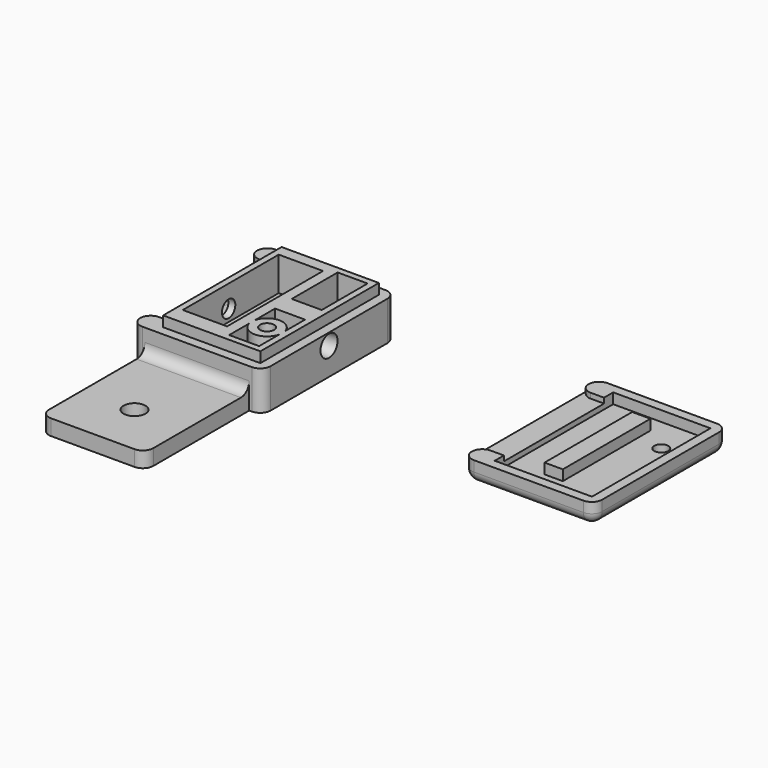
from build123d import *

# Parameters (mm, degrees)
F0_W      = 2
F0_H      = 24
F0_W_2    = 20
F0_H_2    = 25
F1_DEPTH  = 3
F2_W      = 8.5
F2_H      = 26
F2_R      = 1.35
F2_W_2    = 5.75
F2_H_2    = 4
F3_DEPTH  = 4.5
F2_R_2    = 2.1
F4_DEPTH  = 25
F5_W      = 18.65
F5_H      = 28.4
F5_R      = 1.35
F5_W_2    = 8.5
F5_H_2    = 26
F5_W_3    = 5.75
F5_H_3    = 11
F6_DEPTH  = 2
F8_R      = 1.1
F7_R      = 1.1
F9_DEPTH  = 11
F9_TAPER  = -5
F8_W      = 24
F8_H      = 4.5
F10_DEPTH = 4.5
F11_W     = 25
F11_H     = 32
F12_DEPTH = 2
F13_W     = 25
F13_H     = 32
F13_W_2   = 18.65
F13_H_2   = 28.4
F14_DEPTH = 2
F15_W     = 3.5
F15_H     = 26
F16_DEPTH = 2
F15_R     = 1.35
F17_DEPTH = 25
F18_W     = 24
F18_H     = 1
F19_DEPTH = 4.6
F20_R     = 1.99999
F20_2_R   = 1.99999
F21_DEPTH = 2
F22_DEPTH = 1
F23_DEPTH = 3
F24_DEPTH = 2


# Not quite as in the source:
# - a fillet or chamfer is up to 0.001 mm smaller than in the source, because OpenCascade refuses the exact size
# - a feature names something its author has since deleted; it is built from what else it names


with BuildPart() as f1:
    # F0 (on Top) → F1 (new body)
    with BuildSketch(Plane.XY):
        Polygon((-15.3945611045, 29.5401477255), (-40.3945611045, 29.5401477255), (-40.3945611045, -2.4598522745), (-37.8945611045, -2.4598522745), (-17.8945611045, -2.4598522745), (-15.3945611045, -2.4598522745), align=None)
        with Locations((-30.3945611045, 13.5401477255)):
            Rectangle(F0_W, F0_H, mode=Mode.SUBTRACT)
        with Locations((-27.8945611045, -14.9598522745)):
            Rectangle(F0_W_2, F0_H_2)
    extrude(amount=F1_DEPTH)

    # F2 (on face) → F3 (join)
    with BuildSketch(Plane.XY.offset(3)):
        Polygon((-40.3945611045, -2.4598522745), (-37.8945611045, -2.4598522745), (-17.8945611045, -2.4598522745), (-15.3945611045, -2.4598522745), (-15.3945611045, 29.5401477255), (-40.3945611045, 29.5401477255), align=None)
        with Locations((-30.3945611045, 13.5401477255)):
            Rectangle(F2_W, F2_H, mode=Mode.SUBTRACT)
        with BuildLine():
            Line((-18.3945611045, 0.5401477255), (-24.1445611045, 0.5401477255))
            Line((-24.1445611045, 0.5401477255), (-24.1445611045, 5.3791825222))
            ThreePointArc((-24.1445611045, 5.3791825222), (-21.2695611045, 3.0901477255), (-18.3945611045, 5.3791825222))
            Line((-18.3945611045, 5.3791825222), (-18.3945611045, 0.5401477255))
        make_face(mode=Mode.SUBTRACT)
        with Locations((-21.2695611045, 6.0401477255)):
            Circle(F2_R, mode=Mode.SUBTRACT)
        with BuildLine():
            Line((-24.1445611045, 26.5401477255), (-18.3945611045, 26.5401477255))
            Line((-18.3945611045, 26.5401477255), (-18.3945611045, 15.5401477255))
            Line((-18.3945611045, 15.5401477255), (-18.3945611045, 11.5401477255))
            Line((-18.3945611045, 11.5401477255), (-18.3945611045, 6.7011129288))
            ThreePointArc((-18.3945611045, 6.7011129288), (-21.2695611045, 8.9901477255), (-24.1445611045, 6.7011129288))
            Line((-24.1445611045, 6.7011129288), (-24.1445611045, 11.5401477255))
            Line((-24.1445611045, 11.5401477255), (-24.1445611045, 15.5401477255))
            Line((-24.1445611045, 15.5401477255), (-24.1445611045, 26.5401477255))
        make_face(mode=Mode.SUBTRACT)
        with Locations((-21.2695611045, 13.5401477255)):
            Rectangle(F2_W_2, F2_H_2)
    extrude(amount=F3_DEPTH)

    # F2 (on face) → F4 (cut)
    with BuildSketch(Plane.XY.offset(3)):
        with Locations((-27.8945611045, -17.4598522745)):
            Circle(F2_R_2)
    extrude(amount=-F4_DEPTH, mode=Mode.SUBTRACT)

    # F5 (on face) → F6 (join)
    with BuildSketch(Plane.XY.offset(7.5)):
        with Locations((-26.5195611045, 13.5401477255)):
            Rectangle(F5_W, F5_H)
        with BuildLine():
            Line((-18.3945611045, 0.5401477255), (-24.1445611045, 0.5401477255))
            Line((-24.1445611045, 0.5401477255), (-24.1445611045, 5.3791825222))
            ThreePointArc((-24.1445611045, 5.3791825222), (-21.2695611045, 3.0901477255), (-18.3945611045, 5.3791825222))
            Line((-18.3945611045, 5.3791825222), (-18.3945611045, 0.5401477255))
        make_face(mode=Mode.SUBTRACT)
        with Locations((-21.2695611045, 6.0401477255)):
            Circle(F5_R, mode=Mode.SUBTRACT)
        with BuildLine():
            Line((-24.1445611045, 11.5401477255), (-18.3945611045, 11.5401477255))
            Line((-18.3945611045, 11.5401477255), (-18.3945611045, 6.7011129288))
            ThreePointArc((-18.3945611045, 6.7011129288), (-21.2695611045, 8.9901477255), (-24.1445611045, 6.7011129288))
            Line((-24.1445611045, 6.7011129288), (-24.1445611045, 11.5401477255))
        make_face(mode=Mode.SUBTRACT)
        with Locations((-30.3945611045, 13.5401477255)):
            Rectangle(F5_W_2, F5_H_2, mode=Mode.SUBTRACT)
        with Locations((-21.2695611045, 21.0401477255)):
            Rectangle(F5_W_3, F5_H_3, mode=Mode.SUBTRACT)
    extrude(amount=F6_DEPTH)

    # F8 (on face) + F7 (on face) → F9 (cut)
    with BuildSketch(Plane(origin=(-40.3945611045, 0, 0), x_dir=(0, -1, 0), z_dir=(-1, 0, 0))):
        with Locations((-13.5401477255, 5.25)):
            Circle(F8_R)
    with BuildSketch(Plane(origin=(-26.1445611045, 0, 0), x_dir=(0, -1, 0), z_dir=(-1, 0, 0))):
        with Locations((-13.5401477255, 5.25)):
            Circle(F7_R)
    extrude(amount=-F9_DEPTH, taper=F9_TAPER, mode=Mode.SUBTRACT)

    # F8 (on face) → F10 (cut)
    with BuildSketch(Plane(origin=(-40.3945611045, 0, 0), x_dir=(0, -1, 0), z_dir=(-1, 0, 0))):
        with Locations((-13.5401477255, 5.25)):
            Rectangle(F8_W, F8_H)
        with Locations((-13.5401477255, 5.25)):
            Circle(F8_R, mode=Mode.SUBTRACT)
    extrude(amount=-F10_DEPTH, mode=Mode.SUBTRACT)

    # F20 (radius 2 in the source; OpenCascade refuses exactly that, so slightly less here)
    f20_edges = [f1.edges().sort_by_distance(p)[0] for p in [
        (-40.394561, 29.540148, 3.75),
        (-40.394561, -2.459852, 3.75),
        (-40.394561, 13.540148, 3),
        (-40.394561, 1.540148, 5.25),
        (-15.394561, 29.540148, 3.75),
        (-15.394561, -2.459852, 3.75),
        (-27.894561, -2.459852, 3),
        (-17.894561, -27.459852, 1.5),
        (-37.894561, -27.459852, 1.5),
        (-40.394561, 25.540148, 5.25),
        (-35.894561, 1.540148, 5.25),
        (-35.894561, 25.540148, 5.25),
    ]]
    fillet(f20_edges, radius=F20_R)

    # F21 (add): a face of the model
    f21_faces = [f1.faces().sort_by_distance(p)[0] for p in [
        (-30.3945611045, 0.5401477255, 6.25),
    ]]
    extrude(f21_faces, amount=F21_DEPTH)

    # F22 (add): a face of the model
    f22_faces = [f1.faces().sort_by_distance(p)[0] for p in [
        (-30.3945611045, 26.5401477255, 6.25),
    ]]
    extrude(f22_faces, amount=F22_DEPTH)


with BuildPart() as f12:
    # F11 (on Top) → F12 (new body)
    with BuildSketch(Plane.XY):
        with Locations((33.7232563645, 16)):
            Rectangle(F11_W, F11_H)
    extrude(amount=F12_DEPTH)

    # F13 (on face) → F14 (join)
    with BuildSketch(Plane.XY.offset(2)):
        with Locations((33.7232563645, 16)):
            Rectangle(F13_W, F13_H)
        with Locations((35.0982563645, 16)):
            Rectangle(F13_W_2, F13_H_2, mode=Mode.SUBTRACT)
    extrude(amount=F14_DEPTH)

    # F15 (on face) → F16 (join)
    with BuildSketch(Plane.XY.offset(2)):
        with Locations((33.7232563645, 16)):
            Rectangle(F15_W, F15_H)
    extrude(amount=F16_DEPTH)

    # F15 (on face) → F17 (cut)
    with BuildSketch(Plane.XY.offset(2)):
        with Locations((40.3482563645, 23.5)):
            Circle(F15_R)
    extrude(amount=-F17_DEPTH, mode=Mode.SUBTRACT)

    # F18 (on face) → F19 (cut)
    with BuildSketch(Plane(origin=(21.2232563645, 0, 0), x_dir=(0, -1, 0), z_dir=(-1, 0, 0))):
        with Locations((-16, 3.5)):
            Rectangle(F18_W, F18_H)
    extrude(amount=-F19_DEPTH, mode=Mode.SUBTRACT)

    # F20#2 (radius 2 in the source; OpenCascade refuses exactly that, so slightly less here)
    f20_2_edges = [f12.edges().sort_by_distance(p)[0] for p in [
        (21.223256, 0, 2),
        (21.223256, 32, 2),
        (21.223256, 28, 3.5),
        (21.223256, 4, 3.5),
        (46.223256, 0, 2),
        (46.223256, 32, 2),
        (33.723256, 32, 0),
        (46.223256, 16, 0),
        (33.723256, 0, 0),
        (21.223256, 16, 0),
    ]]
    fillet(f20_2_edges, radius=F20_2_R)

    # F23 (cut): a face of the model
    f23_faces = [f12.faces().sort_by_distance(p)[0] for p in [
        (33.7232563645, 3, 3),
    ]]
    extrude(f23_faces, amount=-F23_DEPTH, mode=Mode.SUBTRACT)

    # F24 (cut): a face of the model
    f24_faces = [f12.faces().sort_by_distance(p)[0] for p in [
        (33.7232563645, 29, 3),
    ]]
    extrude(f24_faces, amount=-F24_DEPTH, mode=Mode.SUBTRACT)


solid = Compound([f1.part, f12.part])
